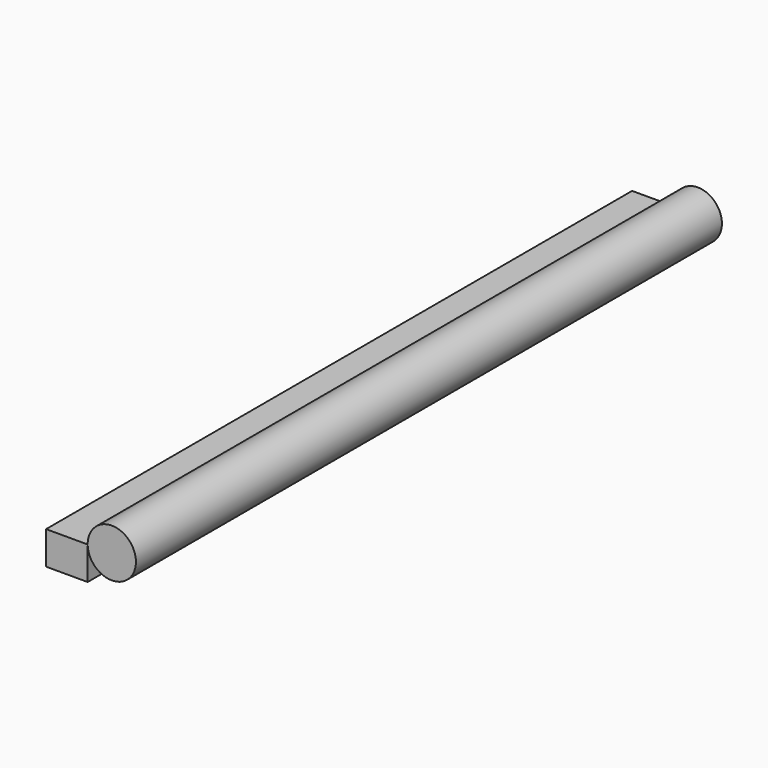
from build123d import *

# Parameters (mm, degrees)
F1_DEPTH = 1143
F0_W     = 64.8966471037
F0_H     = 51.6150052091


with BuildPart() as f1:
    # F0 (on Front) → F1 (new body)
    with BuildSketch(Plane.XZ):
        with BuildLine():
            ThreePointArc((-6.4121966878, 7.5626427671), (31.5047843029, -29.546284868), (68.8849946834, 8.1032812595))
            ThreePointArc((68.8849946834, 8.1032812595), (30.9641318748, 45.7528473871), (-6.4121966878, 7.5626427671))
        make_face()
    extrude(amount=F1_DEPTH)


with BuildPart() as f1b:
    # F0 (on Front) → F1, piece 2 (new body)
    with BuildSketch(Plane.XZ):
        with Locations((-38.8605202396, -18.2448598374)):
            Rectangle(F0_W, F0_H)
    extrude(amount=F1_DEPTH)


solid = Compound([f1.part, f1b.part])
